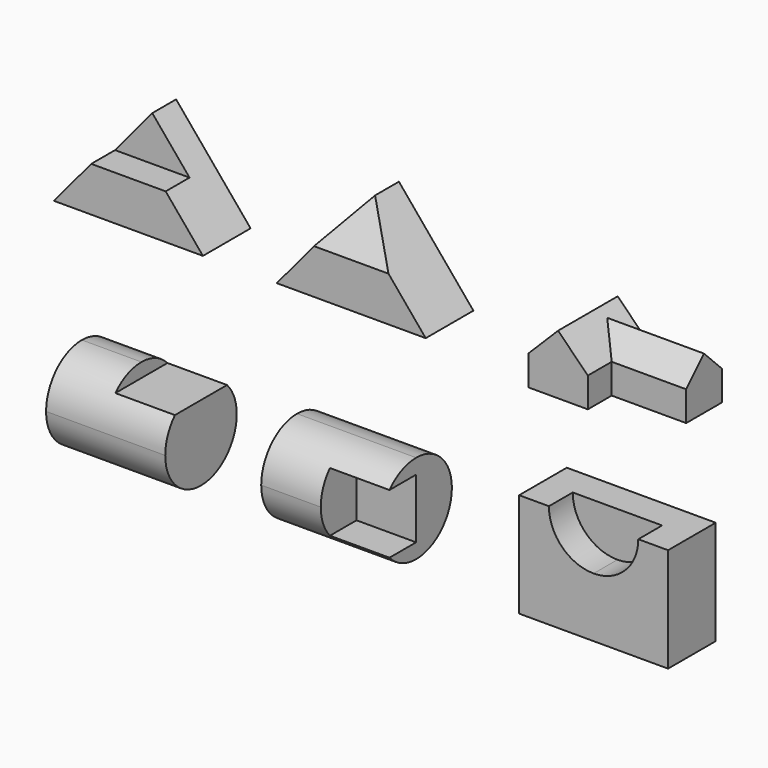
from build123d import *

# Parameters (mm, degrees)
F1_DEPTH  = 101.6
F3_DEPTH  = 50.8
F5_DEPTH  = 101.6
F9_DEPTH  = 76.2
F11_DEPTH = 127
F13_W     = 38.1
F13_H     = 50.8
F14_DEPTH = 177.8
F15_W     = 203.2
F15_H     = 152.4
F16_DEPTH = 152.4
F19_DEPTH = 360.68
F18_W     = 101.6
F18_H     = 24.0481388064
F20_DEPTH = 185.42
F21_W     = 203.2
F21_H     = 152.4
F22_DEPTH = 152.4
F25_DEPTH = 203.2
F26_DEPTH = 101.6
F27_W     = 254
F27_H     = 177.8
F28_DEPTH = 101.6
F30_DEPTH = 50.8


with BuildPart() as f1:
    # F0 (on Front) → F1 (new body)
    with BuildSketch(Plane.XZ):
        Polygon((-127, 0), (0, 0), (127, 0), (63.5, 76.2), (0, 76.2), (-63.5, 76.2), align=None)
        Polygon((0, 76.2), (63.5, 76.2), (0, 152.4), (-63.5, 76.2), align=None)
    extrude(amount=F1_DEPTH)

    # F2 (on face) → F3 (cut)
    with BuildSketch(Plane.XZ.offset(101.6)):
        Polygon((-63.5, 76.2), (0, 76.2), (63.5, 76.2), (0, 152.4), align=None)
    extrude(amount=-F3_DEPTH, mode=Mode.SUBTRACT)


with BuildPart() as f5:
    # F4 (on Front) → F5 (new body)
    with BuildSketch(Plane.XZ):
        Polygon((316.4328755193, 76.2), (252.9328755193, 0), (506.9328755193, 0), (443.4328755193, 76.2), align=None)
        Polygon((379.9328755193, 152.4), (316.4328755193, 76.2), (443.4328755193, 76.2), align=None)
    extrude(amount=F5_DEPTH)

    # F8 (on 3pt) → F9 (cut, symmetric)
    with BuildSketch(Plane.YZ.offset(379.9328755193)):
        Polygon((-50.8, 152.4), (-101.6, 152.4), (-101.6, 76.2), align=None)
    extrude(amount=F9_DEPTH, both=True, mode=Mode.SUBTRACT)


with BuildPart() as f11:
    # F10 (on Front) → F11 (new body)
    with BuildSketch(Plane.XZ):
        Polygon((752.9406986994, 101.6), (752.9406986994, 0), (803.7406986994, 0), (803.7406986994, 50.8), align=None)
        Polygon((702.1406986994, 50.8), (702.1406986994, 0), (752.9406986994, 0), (752.9406986994, 101.6), align=None)
    extrude(amount=F11_DEPTH)

    # F13 (on offset) → F14 (join)
    with BuildSketch(Plane.YZ.offset(930.7406986994)):
        Polygon((-76.2, 50.8), (-38.1, 50.8), (-38.1, 88.9), align=None)
        Polygon((-38.1, 50.8), (0, 50.8), (-38.1, 88.9), align=None)
        with Locations((-19.05, 25.4)):
            Rectangle(F13_W, F13_H)
        with Locations((-57.15, 25.4)):
            Rectangle(F13_W, F13_H)
    extrude(amount=-F14_DEPTH)


with BuildPart() as f16:
    # F15 (on Front) → F16 (new body)
    with BuildSketch(Plane.XZ):
        with Locations((1.7657876015, -286.5948253898)):
            Rectangle(F15_W, F15_H)
    extrude(amount=F16_DEPTH)

    # F17 (on face) → F19 (cut)
    with BuildSketch(Plane.YZ.offset(103.3657876015)):
        with BuildLine():
            ThreePointArc((-152.4, -286.5948253898), (-130.0815367264, -232.7132886634), (-76.2, -210.3948253898))
            Line((-76.2, -210.3948253898), (-152.4, -210.3948253898))
            Line((-152.4, -210.3948253898), (-152.4, -286.5948253898))
        make_face()
        with BuildLine():
            Line((0, -210.3948253898), (-76.2, -210.3948253898))
            ThreePointArc((-76.2, -210.3948253898), (-22.3184632736, -232.7132886634), (0, -286.5948253898))
            Line((0, -286.5948253898), (0, -210.3948253898))
        make_face()
        with BuildLine():
            Line((0, -362.7948253898), (0, -286.5948253898))
            ThreePointArc((0, -286.5948253898), (-22.3184632736, -340.4763621162), (-76.2, -362.7948253898))
            Line((-76.2, -362.7948253898), (0, -362.7948253898))
        make_face()
        with BuildLine():
            ThreePointArc((-76.2, -362.7948253898), (-130.0815367264, -340.4763621162), (-152.4, -286.5948253898))
            Line((-152.4, -286.5948253898), (-152.4, -362.7948253898))
            Line((-152.4, -362.7948253898), (-76.2, -362.7948253898))
        make_face()
    extrude(amount=-F19_DEPTH, mode=Mode.SUBTRACT)

    # F18 (on face) → F20 (cut)
    with BuildSketch(Plane.XZ.offset(152.4)):
        with Locations((52.5657876015, -222.418894793)):
            Rectangle(F18_W, F18_H)
    extrude(amount=-F20_DEPTH, mode=Mode.SUBTRACT)


with BuildPart() as f22:
    # F21 (on Front) → F22 (new body)
    with BuildSketch(Plane.XZ):
        with Locations((368.6252981424, -277.9140620219)):
            Rectangle(F21_W, F21_H)
    extrude(amount=F22_DEPTH)

    # F23 (on face) → F25 (cut)
    with BuildSketch(Plane.YZ.offset(470.2252981424)):
        with BuildLine():
            Line((-152.4, -201.7140620219), (-152.4, -277.9140620219))
            ThreePointArc((-152.4, -277.9140620219), (-130.0815367264, -224.0325252955), (-76.2, -201.7140620219))
            Line((-76.2, -201.7140620219), (-152.4, -201.7140620219))
        make_face()
        with BuildLine():
            ThreePointArc((-76.2, -201.7140620219), (-22.3184632736, -224.0325252955), (0, -277.9140620219))
            Line((0, -277.9140620219), (0, -201.7140620219))
            Line((0, -201.7140620219), (-76.2, -201.7140620219))
        make_face()
        with BuildLine():
            ThreePointArc((0, -277.9140620219), (-22.3184632736, -331.7955987483), (-76.2, -354.1140620219))
            Line((-76.2, -354.1140620219), (0, -354.1140620219))
            Line((0, -354.1140620219), (0, -277.9140620219))
        make_face()
        with BuildLine():
            Line((-152.4, -354.1140620219), (-76.2, -354.1140620219))
            ThreePointArc((-76.2, -354.1140620219), (-130.0815367264, -331.7955987483), (-152.4, -277.9140620219))
            Line((-152.4, -277.9140620219), (-152.4, -354.1140620219))
        make_face()
    extrude(amount=-F25_DEPTH, mode=Mode.SUBTRACT)

    # F24 (on face) → F26 (cut)
    with BuildSketch(Plane.YZ.offset(470.2252981424)):
        with BuildLine():
            Line((-76.2, -227.1140620219), (-132.9961266285, -227.1140620219))
            ThreePointArc((-132.9961266285, -227.1140620219), (-147.383933753, -250.7242187812), (-152.4, -277.9140620219))
            Line((-152.4, -277.9140620219), (-76.2, -277.9140620219))
            Line((-76.2, -277.9140620219), (-76.2, -227.1140620219))
        make_face()
        with BuildLine():
            Line((-76.2, -277.9140620219), (-152.4, -277.9140620219))
            ThreePointArc((-152.4, -277.9140620219), (-147.383933753, -305.1039052626), (-132.9961266285, -328.7140620219))
            Line((-132.9961266285, -328.7140620219), (-76.2, -328.7140620219))
            Line((-76.2, -328.7140620219), (-76.2, -277.9140620219))
        make_face()
    extrude(amount=-F26_DEPTH, mode=Mode.SUBTRACT)


with BuildPart() as f28:
    # F27 (on Front) → F28 (new body)
    with BuildSketch(Plane.XZ):
        with Locations((793.1881248951, -272.8261766908)):
            Rectangle(F27_W, F27_H)
    extrude(amount=F28_DEPTH)

    # F29 (on face) → F30 (cut)
    with BuildSketch(Plane.XZ.offset(101.6)):
        with BuildLine():
            Line((793.1881248951, -260.1261766908), (793.1881248951, -183.9261766908))
            Line((793.1881248951, -183.9261766908), (716.9881248951, -183.9261766908))
            ThreePointArc((716.9881248951, -183.9261766908), (739.3065881687, -237.8077134172), (793.1881248951, -260.1261766908))
        make_face()
        with BuildLine():
            Line((869.3881248951, -183.9261766908), (793.1881248951, -183.9261766908))
            Line((793.1881248951, -183.9261766908), (793.1881248951, -260.1261766908))
            ThreePointArc((793.1881248951, -260.1261766908), (847.0696616215, -237.8077134172), (869.3881248951, -183.9261766908))
        make_face()
    extrude(amount=-F30_DEPTH, mode=Mode.SUBTRACT)


solid = Compound([f1.part, f5.part, f11.part, f16.part, f22.part, f28.part])
